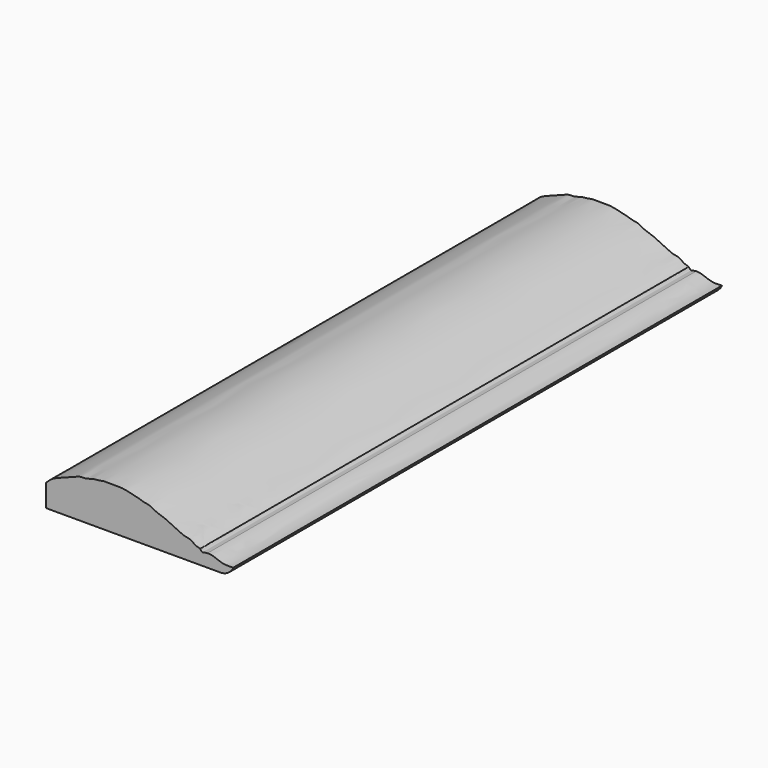
from build123d import *

# Parameters (mm, degrees)
F1_DEPTH    = 215
F2_T1_DEPTH = 237.9128784748


# Not quite as in the source:
# - a fillet or chamfer that OpenCascade refuses, or shapes differently, is made with other operations: its cross-section is extruded or revolved along the edge and cut away or added


with BuildPart() as f1:
    # F0 (on Front) → F1 (new body)
    with BuildSketch(Plane.XZ):
        with BuildLine():
            add(Edge.make_bspline(
                [(-65.4067975488, 7.9), (-64.7446827642, 8.5441405082), (-63.477396389, 9.7770241543), (-61.3556983755, 10.6763060463), (-59.3261192012, 11.536081627), (-57.2882532943, 12.2802882653), (-55.2594103899, 12.9664310821), (-53.2594358742, 13.8360781513), (-51.1660118118, 13.5695464853), (-49.1928290211, 14.5178863994), (-47.1276857108, 14.506671967), (-45.1170711888, 15.0563899138), (-43.075192109, 14.9051977862), (-41.0476544737, 14.9031676075), (-39.0115486283, 15.0022986162), (-36.9779374337, 14.6654074526), (-34.9572495613, 14.1678726088), (-32.91324085, 13.7384022898), (-30.9210670552, 12.9504590852), (-28.7989996539, 12.8276635908), (-26.8826100013, 11.4491985592), (-24.7948716824, 10.8991034099), (-22.7490904289, 10.1024848406), (-20.7688732719, 8.9435573213), (-18.7126441336, 8.148796087), (-16.7299758299, 7.0842785912), (-14.5717633458, 7.0488862609), (-12.7638127336, 5.3273663002), (-11.5660546149, 5.2626631044), (-11.2112825736, 5)],
                knots=[0, 0, 0, 0, 0.0338753916, 0.0650257007, 0.0956580751, 0.1260648577, 0.1564155231, 0.1865884769, 0.21605978, 0.2461084444, 0.2756564169, 0.3053063957, 0.3347521875, 0.3641979794, 0.3936437713, 0.423238481, 0.4530550197, 0.4829374078, 0.513045091, 0.5428174627, 0.574061051, 0.604391979, 0.6349455091, 0.6661890973, 0.6969857938, 0.7276449479, 0.7574937799, 0.7893686126, 0.8147768362, 0.8147768362, 0.8147768362, 0.8147768362], degree=3))
            Line((-65.4067975488, 7.9), (-65.4067975488, 0))
            Line((-65.4067975488, 0), (0.5232024512, 0))
            Line((0.5232024512, 0), (0.5232024512, 3))
            add(Edge.make_bspline(
                [(-8.5667975488, 4.52), (-7.8700649184, 4.5654690193), (-6.5006401691, 4.3350148914), (-4.5552721521, 3.4462995441), (-2.2420579262, 2.8648207953), (-1.1070154242, 2.947469133), (0.5232024512, 3)],
                knots=[0.8743439824, 0.8743439824, 0.8743439824, 0.8743439824, 0.903918966, 0.934321718, 0.9642041061, 1, 1, 1, 1], degree=3))
            add(Edge.make_bspline(
                [(-11.2112825736, 5), (-10.933856182, 4.7946014094), (-10.6523620488, 4.2158777781), (-10.1538388519, 4.2262545919), (-9.192728764, 4.4791515062), (-8.5667975488, 4.52)],
                knots=[0.8147768362, 0.8147768362, 0.8147768362, 0.8147768362, 0.8346456843, 0.847774385, 0.8743439824, 0.8743439824, 0.8743439824, 0.8743439824], degree=3))
        make_face()
    extrude(amount=F1_DEPTH)

    # F2: fillet of radius 5 on 1 edges, made by hand

    # F2_s2 → F2_t1 (cut)
    with BuildSketch(Plane.XZ.offset(-11.4564392374)):
        with BuildLine():
            ThreePointArc((0.5232024512, 3), (-1.3207604562, 0.8166998673), (-4.0593732438, 0))
            Line((-4.0593732438, 0), (0.5232024512, 0))
            Line((0.5232024512, 0), (0.5232024512, 3))
        make_face()
    extrude(amount=F2_T1_DEPTH, mode=Mode.SUBTRACT)


solid = f1.part
